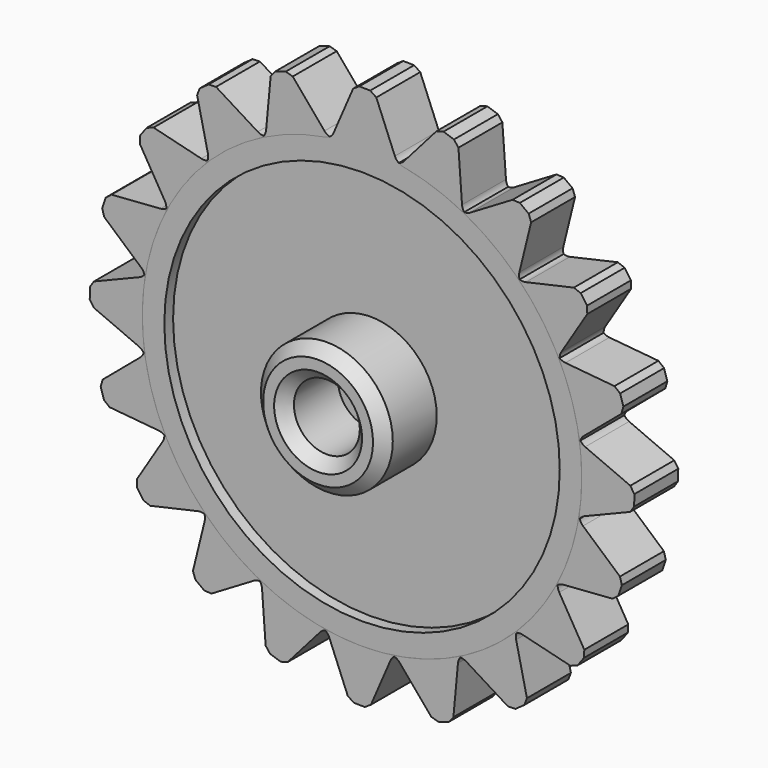
from build123d import *

# Parameters (mm, degrees)
F0_R      = 100
F1_DEPTH  = 25
F3_DEPTH  = 25
F4_R      = 5
F5_SIZE   = 2
F6_COUNT  = 20
F7_R      = 90
F8_DEPTH  = 5
F9_R      = 30
F10_DEPTH = 30
F11_R     = 15
F12_DEPTH = 49
F13_SIZE  = 5


with BuildPart() as f1:
    # F0 (on Front) → F1 (new body)
    with BuildSketch(Plane.XZ):
        Circle(F0_R)
    extrude(amount=F1_DEPTH)

    # F2 (on face) → F3 (join)
    with BuildSketch(Plane.XZ.offset(25)):
        with BuildLine():
            Line((35.2033524134, 118.8919231231), (17.2731788453, 98.4968897609))
            ThreePointArc((17.2731788453, 98.4968897609), (31.8522835064, 94.7915187948), (45.7106344837, 88.941204709))
            Line((45.7106344837, 88.941204709), (43.7345891049, 116.0252176076))
            Line((43.7345891049, 116.0252176076), (35.2033524134, 118.8919231231))
        make_face()
        with BuildLine():
            Line((45.7106344837, 88.941204709), (17.2731788453, 98.4968897609))
            ThreePointArc((17.2731788453, 98.4968897609), (-76.5745319428, -64.3143923064), (100, 0))
            ThreePointArc((100, 0), (85.355326279, 52.1005592658), (45.7106344837, 88.941204709))
        make_face()
    extrude(amount=-F3_DEPTH)

    # F4
    f4_edges = [f1.edges().sort_by_distance(p)[0] for p in [
        (17.273179, -12.5, 98.49689),
        (45.710634, -12.5, 88.941205),
    ]]
    fillet(f4_edges, radius=F4_R)

    # F5
    f5_edges = [f1.edges().sort_by_distance(p)[0] for p in [
        (35.203352, -12.5, 118.891923),
        (43.734589, -12.5, 116.025218),
    ]]
    chamfer(f5_edges, length=F5_SIZE)


with BuildPart() as f6_1:
    # F6: instance of F1
    add(f1.part.rotate(Axis((0, 0, 0), (0, 1, 0)), 1 * 360 / F6_COUNT))


with BuildPart() as f6_2:
    # F6: instance of F1
    add(f1.part.rotate(Axis((0, 0, 0), (0, 1, 0)), 2 * 360 / F6_COUNT))


with BuildPart() as f6_3:
    # F6: instance of F1
    add(f1.part.rotate(Axis((0, 0, 0), (0, 1, 0)), 3 * 360 / F6_COUNT))


with BuildPart() as f6_4:
    # F6: instance of F1
    add(f1.part.rotate(Axis((0, 0, 0), (0, 1, 0)), 4 * 360 / F6_COUNT))


with BuildPart() as f6_5:
    # F6: instance of F1
    add(f1.part.rotate(Axis((0, 0, 0), (0, 1, 0)), 5 * 360 / F6_COUNT))


with BuildPart() as f6_6:
    # F6: instance of F1
    add(f1.part.rotate(Axis((0, 0, 0), (0, 1, 0)), 6 * 360 / F6_COUNT))


with BuildPart() as f6_7:
    # F6: instance of F1
    add(f1.part.rotate(Axis((0, 0, 0), (0, 1, 0)), 7 * 360 / F6_COUNT))


with BuildPart() as f6_8:
    # F6: instance of F1
    add(f1.part.rotate(Axis((0, 0, 0), (0, 1, 0)), 8 * 360 / F6_COUNT))


with BuildPart() as f6_9:
    # F6: instance of F1
    add(f1.part.rotate(Axis((0, 0, 0), (0, 1, 0)), 9 * 360 / F6_COUNT))


with BuildPart() as f6_10:
    # F6: instance of F1
    add(f1.part.rotate(Axis((0, 0, 0), (0, 1, 0)), 10 * 360 / F6_COUNT))


with BuildPart() as f6_11:
    # F6: instance of F1
    add(f1.part.rotate(Axis((0, 0, 0), (0, 1, 0)), 11 * 360 / F6_COUNT))


with BuildPart() as f6_12:
    # F6: instance of F1
    add(f1.part.rotate(Axis((0, 0, 0), (0, 1, 0)), 12 * 360 / F6_COUNT))


with BuildPart() as f6_13:
    # F6: instance of F1
    add(f1.part.rotate(Axis((0, 0, 0), (0, 1, 0)), 13 * 360 / F6_COUNT))


with BuildPart() as f6_14:
    # F6: instance of F1
    add(f1.part.rotate(Axis((0, 0, 0), (0, 1, 0)), 14 * 360 / F6_COUNT))


with BuildPart() as f6_15:
    # F6: instance of F1
    add(f1.part.rotate(Axis((0, 0, 0), (0, 1, 0)), 15 * 360 / F6_COUNT))


with BuildPart() as f6_16:
    # F6: instance of F1
    add(f1.part.rotate(Axis((0, 0, 0), (0, 1, 0)), 16 * 360 / F6_COUNT))


with BuildPart() as f6_17:
    # F6: instance of F1
    add(f1.part.rotate(Axis((0, 0, 0), (0, 1, 0)), 17 * 360 / F6_COUNT))


with BuildPart() as f6_18:
    # F6: instance of F1
    add(f1.part.rotate(Axis((0, 0, 0), (0, 1, 0)), 18 * 360 / F6_COUNT))


with BuildPart() as f6_19:
    # F6: instance of F1
    add(f1.part.rotate(Axis((0, 0, 0), (0, 1, 0)), 19 * 360 / F6_COUNT))


with BuildPart() as f8_tool:
    # F7 (on face) → F8 (new body)
    with BuildSketch(Plane.XZ.offset(25)):
        Circle(F7_R)
    extrude(amount=-F8_DEPTH)


with BuildPart() as f1_1:
    add(f1.part)

    # F8: cut by f8_tool
    add(f8_tool.part, mode=Mode.SUBTRACT)


with BuildPart() as f6_1_1:
    add(f6_1.part)

    # F8: cut by f8_tool
    add(f8_tool.part, mode=Mode.SUBTRACT)


with BuildPart() as f6_2_1:
    add(f6_2.part)

    # F8: cut by f8_tool
    add(f8_tool.part, mode=Mode.SUBTRACT)


with BuildPart() as f6_3_1:
    add(f6_3.part)

    # F8: cut by f8_tool
    add(f8_tool.part, mode=Mode.SUBTRACT)


with BuildPart() as f6_4_1:
    add(f6_4.part)

    # F8: cut by f8_tool
    add(f8_tool.part, mode=Mode.SUBTRACT)


with BuildPart() as f6_5_1:
    add(f6_5.part)

    # F8: cut by f8_tool
    add(f8_tool.part, mode=Mode.SUBTRACT)


with BuildPart() as f6_6_1:
    add(f6_6.part)

    # F8: cut by f8_tool
    add(f8_tool.part, mode=Mode.SUBTRACT)


with BuildPart() as f6_7_1:
    add(f6_7.part)

    # F8: cut by f8_tool
    add(f8_tool.part, mode=Mode.SUBTRACT)


with BuildPart() as f6_8_1:
    add(f6_8.part)

    # F8: cut by f8_tool
    add(f8_tool.part, mode=Mode.SUBTRACT)


with BuildPart() as f6_9_1:
    add(f6_9.part)

    # F8: cut by f8_tool
    add(f8_tool.part, mode=Mode.SUBTRACT)


with BuildPart() as f6_10_1:
    add(f6_10.part)

    # F8: cut by f8_tool
    add(f8_tool.part, mode=Mode.SUBTRACT)


with BuildPart() as f6_11_1:
    add(f6_11.part)

    # F8: cut by f8_tool
    add(f8_tool.part, mode=Mode.SUBTRACT)


with BuildPart() as f6_12_1:
    add(f6_12.part)

    # F8: cut by f8_tool
    add(f8_tool.part, mode=Mode.SUBTRACT)


with BuildPart() as f6_13_1:
    add(f6_13.part)

    # F8: cut by f8_tool
    add(f8_tool.part, mode=Mode.SUBTRACT)


with BuildPart() as f6_14_1:
    add(f6_14.part)

    # F8: cut by f8_tool
    add(f8_tool.part, mode=Mode.SUBTRACT)


with BuildPart() as f6_15_1:
    add(f6_15.part)

    # F8: cut by f8_tool
    add(f8_tool.part, mode=Mode.SUBTRACT)


with BuildPart() as f6_16_1:
    add(f6_16.part)

    # F8: cut by f8_tool
    add(f8_tool.part, mode=Mode.SUBTRACT)


with BuildPart() as f6_17_1:
    add(f6_17.part)

    # F8: cut by f8_tool
    add(f8_tool.part, mode=Mode.SUBTRACT)


with BuildPart() as f6_18_1:
    add(f6_18.part)

    # F8: cut by f8_tool
    add(f8_tool.part, mode=Mode.SUBTRACT)


with BuildPart() as f6_19_1:
    add(f6_19.part)

    # F8: cut by f8_tool
    add(f8_tool.part, mode=Mode.SUBTRACT)


with BuildPart() as f10:
    # F9 (on face) → F10 (new body)
    with BuildSketch(Plane.XZ.offset(20)):
        Circle(F9_R)
    extrude(amount=F10_DEPTH)

    # F11 (on face) → F12 (cut)
    with BuildSketch(Plane.XZ.offset(50)):
        Circle(F11_R)
    extrude(amount=-F12_DEPTH, mode=Mode.SUBTRACT)

    # F13
    f13_edges = [f10.edges().sort_by_distance(p)[0] for p in [
        (-30, -50, 0),
        (-15, -50, 0),
    ]]
    chamfer(f13_edges, length=F13_SIZE)


solid = Compound([f1_1.part, f6_1_1.part, f6_2_1.part, f6_3_1.part, f6_4_1.part, f6_5_1.part, f6_6_1.part, f6_7_1.part, f6_8_1.part, f6_9_1.part, f6_10_1.part, f6_11_1.part, f6_12_1.part, f6_13_1.part, f6_14_1.part, f6_15_1.part, f6_16_1.part, f6_17_1.part, f6_18_1.part, f6_19_1.part, f10.part])
